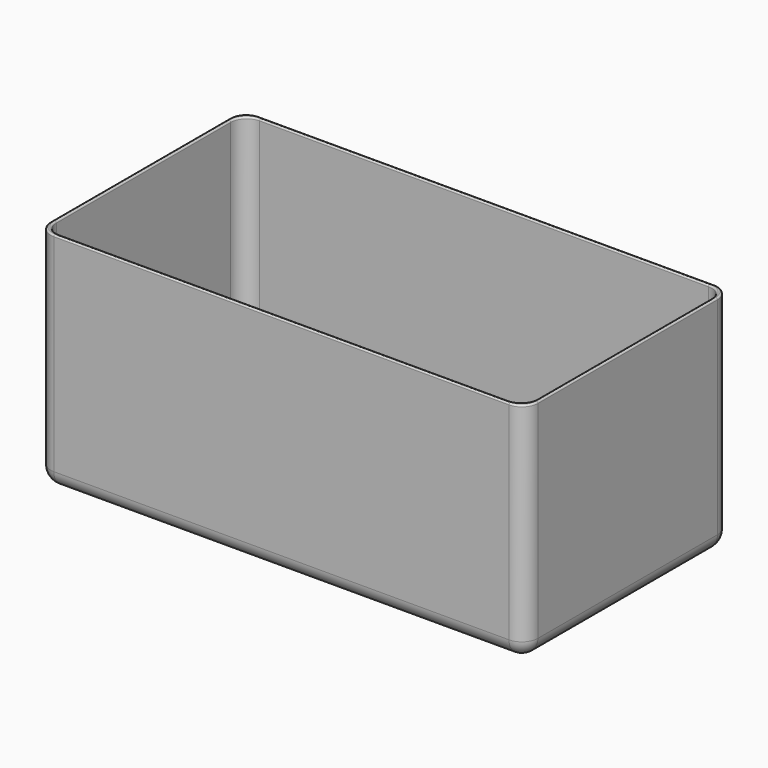
from build123d import *

# Parameters (mm, degrees)
F0_W     = 152
F0_H     = 80
F1_DEPTH = 70
F2_W     = 150
F2_H     = 78
F3_DEPTH = 69
F4_R     = 5
F5_R     = 5
F6_R     = 0.49999


# Not quite as in the source:
# - a fillet or chamfer is up to 0.001 mm smaller than in the source, because OpenCascade refuses the exact size


with BuildPart() as f1:
    # F0 (on Top) → F1 (new body)
    with BuildSketch(Plane.XY):
        Rectangle(F0_W, F0_H)
    extrude(amount=F1_DEPTH)

    # F2 (on face) → F3 (cut)
    with BuildSketch(Plane.XY.offset(70)):
        Rectangle(F2_W, F2_H)
    extrude(amount=-F3_DEPTH, mode=Mode.SUBTRACT)

    # F4
    f4_edges = [f1.edges().sort_by_distance(p)[0] for p in [
        (-75, 39, 35.5),
        (-75, -39, 35.5),
        (75, -39, 35.5),
        (75, 39, 35.5),
        (0, -39, 1),
        (75, 0, 1),
        (0, 39, 1),
        (-75, 0, 1),
        (0, -40, 0),
    ]]
    fillet(f4_edges, radius=F4_R)

    # F5
    f5_edges = [f1.edges().sort_by_distance(p)[0] for p in [
        (0, -40, 5),
        (-76, -40, 37.5),
        (-76, 40, 35),
        (76, 2.5, 0),
        (76, 40, 35),
        (0, 40, 0),
    ]]
    fillet(f5_edges, radius=F5_R)

    # F6 (radius 0.5 in the source; OpenCascade refuses exactly that, so slightly less here)
    f6_edges = [f1.edges().sort_by_distance(p)[0] for p in [
        (0, 40, 70),
        (0, -39, 70),
        (0, 39, 70),
        (75, 0, 70),
        (-73.535534, -37.535534, 70),
        (-75, 0, 70),
        (73.535534, 37.535534, 70),
        (0, -40, 70),
        (76, 0, 70),
        (74.535534, -38.535534, 70),
        (-76, 0, 70),
        (-74.535534, -38.535534, 70),
        (-74.535534, 38.535534, 70),
        (74.535534, 38.535534, 70),
        (73.535534, -37.535534, 70),
        (-73.535534, 37.535534, 70),
    ]]
    fillet(f6_edges, radius=F6_R)


solid = f1.part
